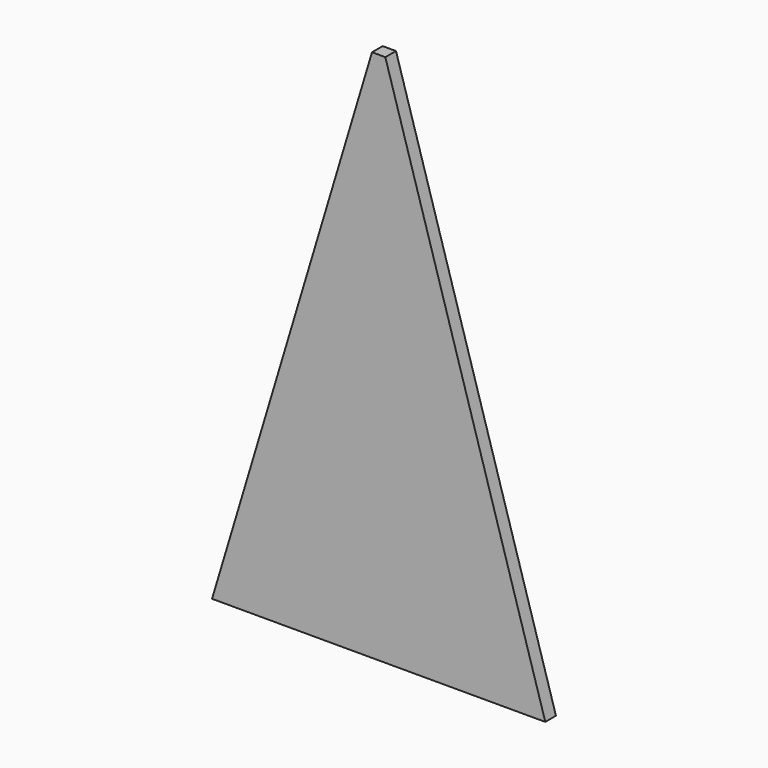
from build123d import *

# Parameters (mm, degrees)
F2_W     = 500
F2_H     = 800
F3_DEPTH = 20
F4_SIZE2 = 799.99999
F4_SIZE  = 239.99999


# Not quite as in the source:
# - a fillet or chamfer is up to 0.001 mm smaller than in the source, because OpenCascade refuses the exact size


with BuildPart() as f3:
    # F2 (on Front) → F3 (new body)
    with BuildSketch(Plane.XZ):
        with Locations((0, 400)):
            Rectangle(F2_W, F2_H)
    extrude(amount=F3_DEPTH)

    # F4 (size 240 and 800 in the source; OpenCascade refuses exactly that, so slightly less here)
    f4_edges = [f3.edges().sort_by_distance(p)[0] for p in [
        (250, -10, 800),
        (-250, -10, 800),
    ]]
    f4_side = f3.faces().sort_by_distance((0, -10, 800))[0]
    chamfer(f4_edges, length=F4_SIZE, length2=F4_SIZE2, reference=f4_side)


solid = f3.part
